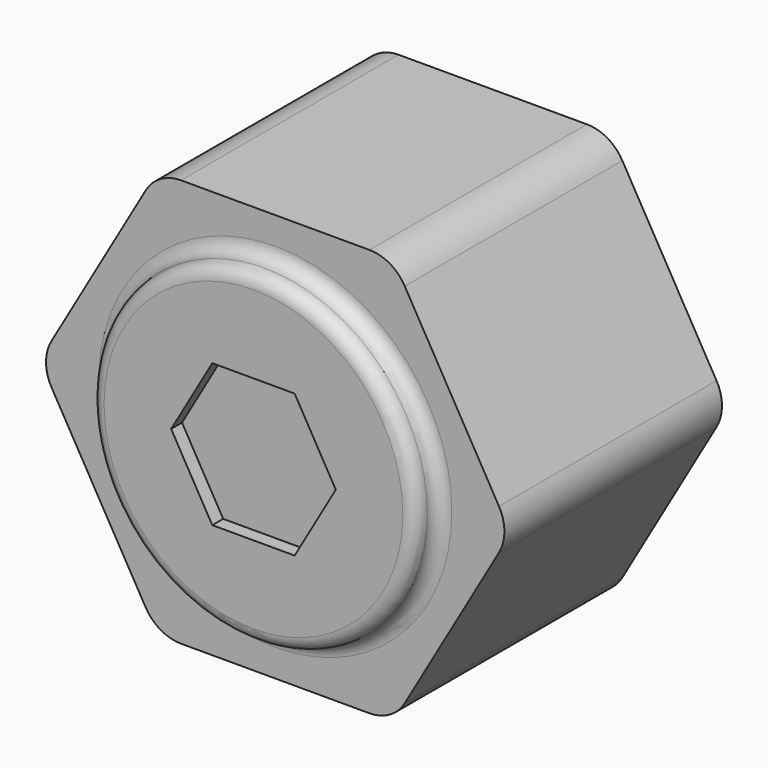
from build123d import *

# Parameters (mm, degrees)
F0_R     = 10
F1_DEPTH = 20
F2_R     = 11.9866247271
F3_DEPTH = 2
F4_R     = 0.99999
F6_DEPTH = 1


# Not quite as in the source:
# - a fillet or chamfer is up to 0.001 mm smaller than in the source, because OpenCascade refuses the exact size


with BuildPart() as f1:
    # F0 (on Front) → F1 (new body)
    with BuildSketch(Plane.XZ):
        with BuildLine():
            Line((6.9282032303, 15), (-6.9282032303, 15))
            ThreePointArc((-6.9282032303, 15), (-8.4282032303, 14.5980762114), (-9.5262794416, 13.5))
            Line((-9.5262794416, 13.5), (-16.4544826719, 1.5))
            ThreePointArc((-16.4544826719, 1.5), (-16.8564064606, 0), (-16.4544826719, -1.5))
            Line((-16.4544826719, -1.5), (-9.5262794416, -13.5))
            ThreePointArc((-9.5262794416, -13.5), (-8.4282032303, -14.5980762114), (-6.9282032303, -15))
            Line((-6.9282032303, -15), (6.9282032303, -15))
            ThreePointArc((6.9282032303, -15), (8.4282032303, -14.5980762114), (9.5262794416, -13.5))
            Line((9.5262794416, -13.5), (16.4544826719, -1.5))
            ThreePointArc((16.4544826719, -1.5), (16.8564064606, 0), (16.4544826719, 1.5))
            Line((16.4544826719, 1.5), (9.5262794416, 13.5))
            ThreePointArc((9.5262794416, 13.5), (8.4282032303, 14.5980762114), (6.9282032303, 15))
        make_face()
        Circle(F0_R, mode=Mode.SUBTRACT)
    extrude(amount=F1_DEPTH)

    # F2 (on face) → F3 (join)
    with BuildSketch(Plane.XZ.offset(20)):
        Circle(F2_R)
    extrude(amount=F3_DEPTH)

    # F4 (radius 1 in the source; OpenCascade refuses exactly that, so slightly less here)
    f4_edges = [f1.edges().sort_by_distance(p)[0] for p in [
        (-11.986625, -22, 0),
        (-11.986625, -20, 0),
    ]]
    fillet(f4_edges, radius=F4_R)

    # F5 (on face) → F6 (cut)
    with BuildSketch(Plane.XZ.offset(22)):
        Polygon((3.027519893, 5.2438182756), (-3.027519893, 5.2438182756), (-6.055039786, 0), (-3.027519893, -5.2438182756), (3.027519893, -5.2438182756), (6.055039786, 0), align=None)
    extrude(amount=-F6_DEPTH, mode=Mode.SUBTRACT)


solid = f1.part
